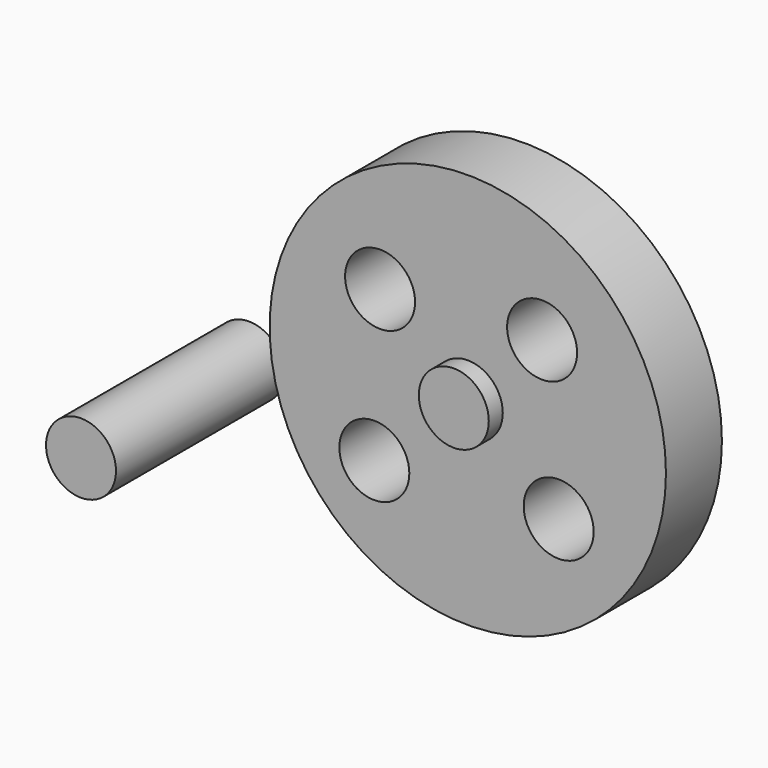
from build123d import *

# Parameters (mm, degrees)
F0_R     = 71.9356029279
F0_R_2   = 12.7
F1_DEPTH = 25.4
F3_DEPTH = 31.75
F4_DEPTH = 76.2


# Not quite as in the source:
# - the program builds the solid bodies; features that only make, move or delete a surface that nothing else refers to are left out


with BuildPart() as f1:
    # F0 (on Front) → F1 (new body)
    with BuildSketch(Plane.XZ):
        Circle(F0_R)
        with Locations((-33.9307952672, -30.3383674473)):
            Circle(F0_R_2, mode=Mode.SUBTRACT)
        with Locations((-31.8473428488, 25.0476300716)):
            Circle(F0_R_2, mode=Mode.SUBTRACT)
        Circle(F0_R_2, mode=Mode.SUBTRACT)
        with Locations((33.0006089061, -27.3112040013)):
            Circle(F0_R_2, mode=Mode.SUBTRACT)
        with Locations((26.9748345017, 27.9723200947)):
            Circle(F0_R_2, mode=Mode.SUBTRACT)
        Circle(F0_R_2)
    extrude(amount=F1_DEPTH)


with BuildPart() as f3:
    # F0 (on Front) → F3 (new body)
    with BuildSketch(Plane.XZ):
        Circle(F0_R_2)
    extrude(amount=F3_DEPTH)


with BuildPart() as f4:
    # F0 (on Front) → F4 (new body)
    with BuildSketch(Plane.XZ):
        with Locations((-99.7780840844, -30.3383674473)):
            Circle(F0_R_2)
    extrude(amount=F4_DEPTH)


solid = Compound([f1.part, f3.part, f4.part])
